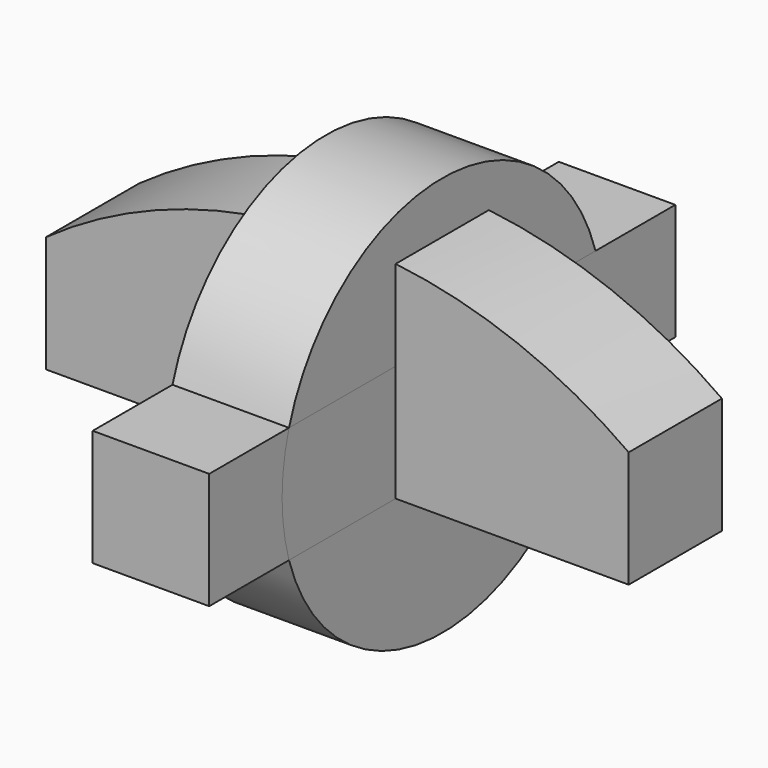
from build123d import *

# Parameters (mm, degrees)
F0_W     = 127
F0_H     = 25.4
F2_DEPTH = 12.7
F3_DEPTH = 12.7
F4_DEPTH = 12.7
F5_DEPTH = 12.7
F6_DEPTH = 12.7
F7_DEPTH = 12.7
F8_DEPTH = 12.7


with BuildPart() as f2:
    # F0 (on Front) → F2 (new body, symmetric)
    with BuildSketch(Plane.XZ):
        Rectangle(F0_W, F0_H)
    extrude(amount=F2_DEPTH, both=True)

    # F0 (on Front) → F4 (join, symmetric)
    with BuildSketch(Plane.XZ):
        with BuildLine():
            ThreePointArc((63.5, 12.7), (0, 33.089700587), (-63.5, 12.7))
            Line((-63.5, 12.7), (63.5, 12.7))
        make_face()
    extrude(amount=F4_DEPTH, both=True)

    # F1 (on Right) → F5 (join, symmetric)
    with BuildSketch(Plane.YZ):
        with BuildLine():
            ThreePointArc((41.7586787839, 12.7), (0, 43.6471906745), (-41.7586787839, 12.7))
            Line((-41.7586787839, 12.7), (41.7586787839, 12.7))
        make_face()
    extrude(amount=F5_DEPTH, both=True)


with BuildPart() as f3:
    # F1 (on Right) → F3 (new body, symmetric)
    with BuildSketch(Plane.YZ):
        with BuildLine():
            Line((-41.7586787839, 12.7), (-63.5, 12.7))
            Line((-63.5, 12.7), (-63.5, -12.7))
            Line((-63.5, -12.7), (-41.7586787839, -12.7))
            ThreePointArc((-41.7586787839, -12.7), (-43.6471906745, 0), (-41.7586787839, 12.7))
        make_face()
    extrude(amount=F3_DEPTH, both=True)


with BuildPart() as f6:
    # F1 (on Right) → F6 (new body, symmetric)
    with BuildSketch(Plane.YZ):
        with BuildLine():
            Line((41.7586787839, 12.7), (-41.7586787839, 12.7))
            ThreePointArc((-41.7586787839, 12.7), (-43.6471906745, 0), (-41.7586787839, -12.7))
            Line((-41.7586787839, -12.7), (41.7586787839, -12.7))
            ThreePointArc((41.7586787839, -12.7), (43.1724812177, -6.4198223722), (43.6471906745, 0))
            ThreePointArc((43.6471906745, 0), (43.1724812177, 6.4198223722), (41.7586787839, 12.7))
        make_face()
    extrude(amount=F6_DEPTH, both=True)

    # F1 (on Right) → F8 (join, symmetric)
    with BuildSketch(Plane.YZ):
        with BuildLine():
            Line((63.5, 12.7), (41.7586787839, 12.7))
            ThreePointArc((41.7586787839, 12.7), (43.1724812177, 6.4198223722), (43.6471906745, 0))
            ThreePointArc((43.6471906745, 0), (43.1724812177, -6.4198223722), (41.7586787839, -12.7))
            Line((41.7586787839, -12.7), (63.5, -12.7))
            Line((63.5, -12.7), (63.5, 12.7))
        make_face()
    extrude(amount=F8_DEPTH, both=True)


with BuildPart() as f7:
    # F1 (on Right) → F7 (new body, symmetric)
    with BuildSketch(Plane.YZ):
        with BuildLine():
            Line((41.7586787839, -12.7), (-41.7586787839, -12.7))
            ThreePointArc((-41.7586787839, -12.7), (0, -43.6471906745), (41.7586787839, -12.7))
        make_face()
    extrude(amount=F7_DEPTH, both=True)


solid = Compound([f2.part, f3.part, f6.part, f7.part])
